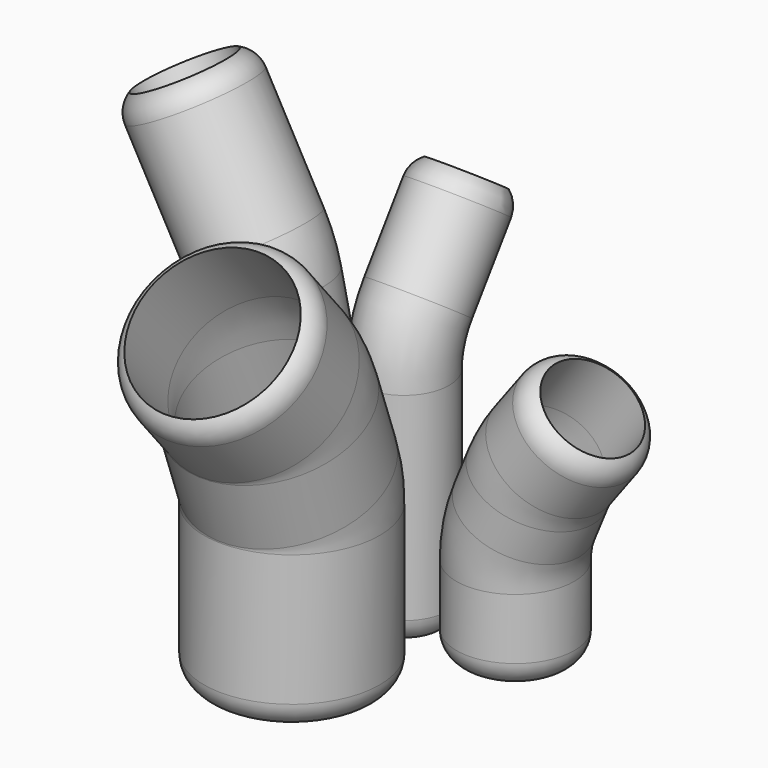
from build123d import *

# Parameters (mm, degrees)
F1_R       = 8.9913396213
F1_R_2     = 7.079086412
F4_R       = 17.5065402818
F4_R_2     = 14.9658997185
F6_T       = -2.54
F8_R       = 11.8315822462
F8_R_2     = 9.4670155796
F10_T      = -2.54
F12_R      = 11.7472705606
F12_R_2    = 9.6747261676
F14_4_F1_R = 5.08
F15_T      = -2.54


# Not quite as in the source:
# - a fillet or chamfer that OpenCascade refuses, or shapes differently, is made with other operations: its cross-section is extruded or revolved along the edge and cut away or added


with BuildPart() as f2:
    # F2: sweep along a path in F0
    with BuildLine(Plane.YZ) as f2_path:
        Line((0, 0), (0, 43.4422037083))
        ThreePointArc((0, 43.4422037083), (0.8953617148, 49.2138246881), (3.4972817569, 54.4429061972))
        Line((3.4972817569, 54.4429061972), (15.5269746691, 71.4504040915))
    # F1 (on Top) → F2 (sweep)
    with BuildSketch(Plane.XY):
        Circle(F1_R)
        Circle(F1_R_2, mode=Mode.SUBTRACT)
    sweep(path=f2_path.line)

    # F14: fillet of radius 5.08 on 7 edges, made by hand

    # F14_s1 → F14_t2 (revolve, cut)
    with BuildSketch(Plane.XZ):
        with BuildLine():
            ThreePointArc((8.9913396213, 3.9713700747), (8.4883776208, 1.7674818852), (7.079086412, 0))
            Line((7.079086412, 0), (8.9913396213, 0))
            Line((8.9913396213, 0), (8.9913396213, 3.9713700747))
        make_face()
    revolve(axis=Axis((0, 0, 0), (0, 0, 1)), mode=Mode.SUBTRACT)

    # F14_s3 → F14_t4 (revolve, cut)
    with BuildSketch(Plane(origin=(0, -23.3361155073, 16.5060319315), x_dir=(1, 0, 0), z_dir=(0, -0.8164156558, 0.5774646976))):
        with BuildLine():
            ThreePointArc((8.9913396213, 63.3281381711), (8.4883776208, 65.5320263605), (7.079086412, 67.2995082457))
            Line((7.079086412, 67.2995082457), (8.9913396213, 67.2995082457))
            Line((8.9913396213, 67.2995082457), (8.9913396213, 63.3281381711))
        make_face()
    revolve(axis=Axis((0, 15.5269746691, 71.4504040915), (0, 0.5774646976, 0.8164156558)), mode=Mode.SUBTRACT)


with BuildPart() as f5:
    # F5: sweep along a path in F3
    with BuildLine(Plane.YZ) as f5_path:
        Line((-27.1323081106, 0), (-27.1323081106, 31.2606439181))
        ThreePointArc((-27.1323081106, 31.2606439181), (-27.4133513821, 34.5208223371), (-28.2481887745, 37.6848064035))
        Line((-28.2481887745, 37.6848064035), (-32.9213116109, 50.7306069746))
        ThreePointArc((-32.9213116109, 50.7306069746), (-34.317361824, 53.7613252226), (-36.2208164308, 56.5019583349))
        Line((-36.2208164308, 56.5019583349), (-47.0485761762, 69.4952681661))
    # F4 (on Top) → F5 (sweep)
    with BuildSketch(Plane.XY):
        with Locations((0, -27.9171578586)):
            Circle(F4_R)
        with Locations((0, -27.9171578586)):
            Circle(F4_R_2, mode=Mode.SUBTRACT)
        with Locations((0, -27.9171578586)):
            Circle(F4_R_2)
    sweep(path=f5_path.line)

    # F6
    f6_openings = [f5.faces().sort_by_distance(p)[0] for p in [
        (0, -47.651514, 68.99282),
    ]]
    offset(amount=F6_T, openings=f6_openings)

    # F14#2: fillet of radius 5.08 on 11 edges, made by hand

    # F14_2_s1 → F14_2_t2 (revolve, cut)
    with BuildSketch(Plane.XZ.offset(27.9171578586)):
        with BuildLine():
            ThreePointArc((12.4265402818, 0), (16.0186427302, 1.4878975516), (17.5065402818, 5.08))
            Line((17.5065402818, 5.08), (17.5065402818, 0))
            Line((17.5065402818, 0), (12.4265402818, 0))
        make_face()
    revolve(axis=Axis((0, -27.9171578586, 0), (0, 0, 1)), mode=Mode.SUBTRACT)

    # F14_2_s3 → F14_2_t4 (revolve, cut)
    with BuildSketch(Plane(origin=(0, 5.8086938174, 4.8405788754), x_dir=(1, 0, 0), z_dir=(0, -0.7682212344, -0.6401844538))):
        with BuildLine():
            ThreePointArc((17.5065402818, 79.1080986911), (16.825949333, 81.6480986911), (14.9665402818, 83.5075077423))
            Line((14.9665402818, 83.5075077423), (17.5065402818, 83.5075077423))
            Line((17.5065402818, 83.5075077423), (17.5065402818, 79.1080986911))
        make_face()
    revolve(axis=Axis((0, -47.6515144184, 68.9928195588), (0, -0.6401844538, 0.7682212344)), mode=Mode.SUBTRACT)


with BuildPart() as f9:
    # F9: sweep along a path in F7
    with BuildLine(Plane.XZ) as f9_path:
        Line((-20.9117194342, 0), (-20.9117194342, 22.0476153873))
        ThreePointArc((-20.9117194342, 22.0476153873), (-21.0588302623, 24.7773751701), (-21.498458684, 27.4755146992))
        Line((-21.498458684, 27.4755146992), (-26.5181254074, 50.422568823))
        ThreePointArc((-26.5181254074, 50.422568823), (-27.5664717226, 53.9606519945), (-29.1164119458, 57.3094947541))
        Line((-29.1164119458, 57.3094947541), (-42.8272224963, 82.0427164435))
    # F8 (on Top) → F9 (sweep)
    with BuildSketch(Plane.XY):
        with Locations((-21.8732375652, 0)):
            Circle(F8_R)
        with Locations((-21.8732375652, 0)):
            Circle(F8_R_2, mode=Mode.SUBTRACT)
        with Locations((-21.8732375652, 0)):
            Circle(F8_R_2)
    sweep(path=f9_path.line)

    # F10
    f10_openings = [f9.faces().sort_by_distance(p)[0] for p in [
        (-43.668171, 0, 81.576538),
    ]]
    offset(amount=F10_T, openings=f10_openings)

    # F14#3: fillet of radius 5.08 on 11 edges, made by hand

    # F14_3_s1 → F14_3_t2 (revolve, cut)
    with BuildSketch(Plane.XZ):
        with BuildLine():
            ThreePointArc((-15.1226210044, -0.0004), (-11.5295528705, 1.4878975516), (-10.0412553189, 5.0809656854))
            Line((-10.0412553189, 5.0809656854), (-9.5331187504, 5.0809656854))
            ThreePointArc((-9.5331187504, 5.0809656854), (-9.5335187504, 2.5404828427), (-9.5335187504, 0))
            Line((-9.5335187504, 0), (-10.0416553189, -0.5081365685))
            ThreePointArc((-10.0416553189, -0.5081365685), (-12.5821381617, -0.5081365685), (-15.1226210044, -0.5085365685))
            Line((-15.1226210044, -0.5085365685), (-15.1226210044, -0.0004))
        make_face()
    revolve(axis=Axis((-21.8732375652, 0, 0), (0, 0, 1)), mode=Mode.SUBTRACT)

    # F14_3_s3 → F14_3_t4 (revolve, cut)
    with BuildSketch(Plane.XZ):
        with BuildLine():
            ThreePointArc((-31.186596544, 83.4648708666), (-33.0135796202, 85.3567584566), (-35.5416973926, 86.0818283444))
            Line((-35.5416973926, 86.0818283444), (-35.5327885497, 86.5898868103))
            ThreePointArc((-35.5327885497, 86.5898868103), (-34.677230936, 87.1416370886), (-33.5665697026, 87.7573298579))
            Line((-33.5665697026, 87.7573298579), (-32.8757880566, 87.5592736483))
            ThreePointArc((-32.8757880566, 87.5592736483), (-31.8091577575, 85.6351566494), (-30.7421776162, 83.7112335847))
            Line((-30.7421776162, 83.7112335847), (-31.186596544, 83.4648708666))
        make_face()
    revolve(axis=Axis((-43.6681713342, 0, 81.5765381856), (-0.4848356395, 0, 0.8746052839)), mode=Mode.SUBTRACT)


with BuildPart() as f13:
    # F13: sweep along a path in F11
    with BuildLine(Plane.XZ) as f13_path:
        Line((20.3802976757, 0), (20.3802976757, 17.1920623273))
        ThreePointArc((20.3802976757, 17.1920623273), (20.8658789176, 22.1349094772), (22.3040565692, 26.8887681343))
        Line((22.3040565692, 26.8887681343), (25.0384157544, 33.5087973258))
        ThreePointArc((25.0384157544, 33.5087973258), (26.4184204613, 36.3387166417), (28.1379329132, 38.9761648884))
        Line((28.1379329132, 38.9761648884), (36.1287072301, 49.713768065))
    # F12 (on Top) → F13 (sweep)
    with BuildSketch(Plane.XY):
        with Locations((22.1610423177, 0)):
            Circle(F12_R)
        with Locations((22.1610423177, 0)):
            Circle(F12_R_2, mode=Mode.SUBTRACT)
        with Locations((22.1610423177, 0)):
            Circle(F12_R_2)
    sweep(path=f13_path.line)

    # F14#4: fillet of radius 5.08 on 9 edges, made by hand

    # F14_4_f1
    f14_4_f1_edges = [f13.edges().sort_by_distance(p)[0] for p in [
        (10.4137717571, 0, 0),
    ]]
    fillet(f14_4_f1_edges, radius=F14_4_F1_R)

    # F15
    f15_openings = [f13.faces().sort_by_distance(p)[0] for p in [
        (37.55728, 0, 48.650644),
    ]]
    offset(amount=F15_T, openings=f15_openings)

    # F16: fillet of radius 5.08 on 3 edges, made by hand

    # F16_s1 → F16_t2 (revolve, cut)
    with BuildSketch(Plane.XZ):
        with BuildLine():
            ThreePointArc((44.3548359588, 38.1080452757), (45.3252506231, 40.5520377918), (44.9436581166, 43.1538047296))
            Line((44.9436581166, 43.1538047296), (46.9813305114, 41.6373973926))
            Line((46.9813305114, 41.6373973926), (44.3548359588, 38.1080452757))
        make_face()
    revolve(axis=Axis((37.5572797495, 0, 48.6506443483), (0.5970107626, 0, 0.8022332263)), mode=Mode.SUBTRACT)


solid = Compound([f2.part, f5.part, f9.part, f13.part])
